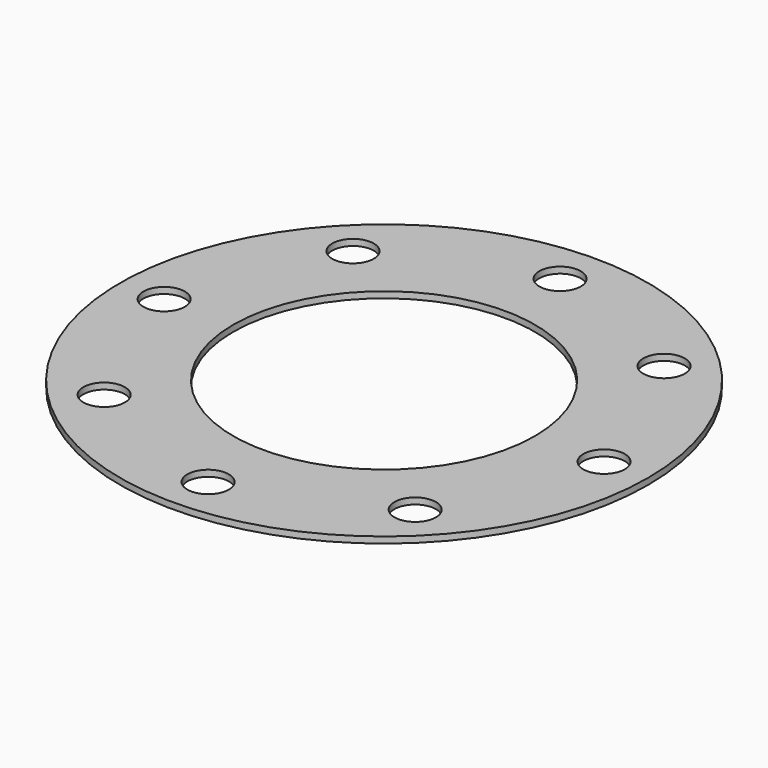
from build123d import *

# Parameters (mm, degrees)
F0_R     = 42
F0_R_2   = 24
F1_DEPTH = 1
F2_D     = 6.6
F2_DEPTH = 12
F2_TIP   = 1.9828400428


# Not quite as in the source:
# - a feature names something its author has since deleted; it is built from what else it names


with BuildPart() as f1:
    # F0 (on Top) → F1 (new body)
    with BuildSketch(Plane.XY):
        Circle(F0_R)
        Circle(F0_R_2, mode=Mode.SUBTRACT)
    extrude(amount=F1_DEPTH)

    # F2
    with Locations(Plane(origin=(0, 0, 0), x_dir=(1, 0, 0), z_dir=(0, 0, -1))):
        with Locations((-24.7487373415, 24.7487373415), (0, 35), (24.7487373415, 24.7487373415), (35, 0), (24.7487373415, -24.7487373415), (0, -35), (-24.7487373415, -24.7487373415), (-35, 0)):
            Hole(F2_D / 2, depth=F2_DEPTH)
            with Locations((0, 0, -(F2_DEPTH + F2_TIP / 2))):  # 118° drill point
                Cone(0, F2_D / 2, F2_TIP, mode=Mode.SUBTRACT)


solid = f1.part
